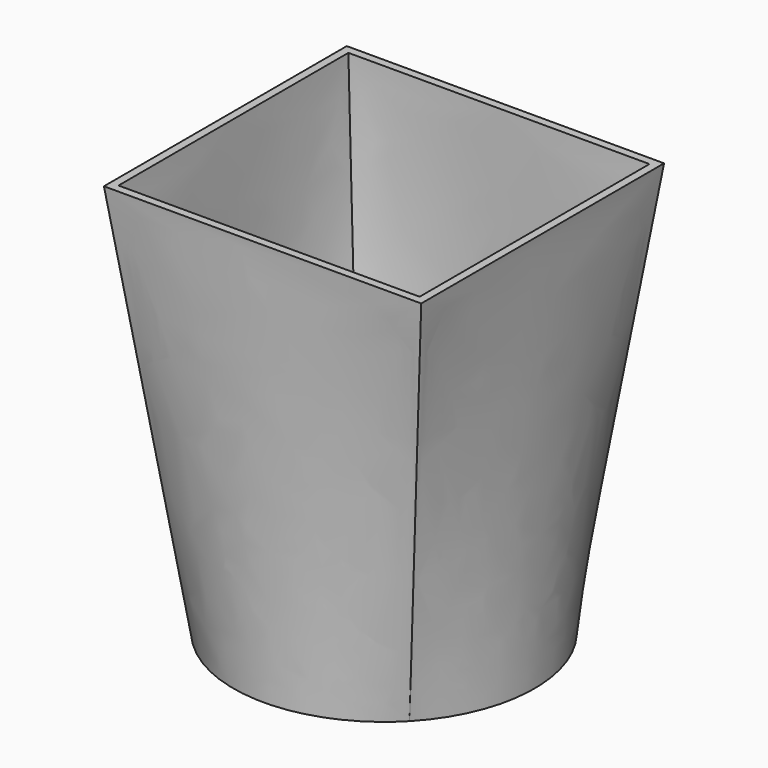
from build123d import *

# Parameters (mm, degrees)
F2_W = 99.9139621854
F2_H = 95.5784469843
F4_T = 2.54


# Not quite as in the source:
# - the arcs of a loft's sections are written as splines that run evenly, so that the points pair up as in the source's solid
# - a shell that OpenCascade refuses in one call is made with other operations: the cavity is built on its own and cut out


with BuildPart() as f3:
    # F2 (on offset) → F3 section 0
    with BuildSketch(Plane.XY.offset(127)):
        Rectangle(F2_W, F2_H)
    # F0 (on Top) → F3 section 1
    with BuildSketch(Plane.XY):
        with BuildLine():
            add(Edge.make_bspline(
                [(34.2488721695, -32.7627284648), (36.3931877331, -30.5211450231), (38.3166790346, -28.0684255821), (41.6482828465, -22.8347310657), (43.0563129764, -20.0538854036), (45.3028578067, -14.2707911992), (46.1413169567, -11.2686856553), (47.2164693474, -5.1584328302), (47.4531360028, -2.0504366369), (47.3155784505, 4.1521612197), (46.9413576443, 7.2466095116), (45.5963764086, 13.3031900424), (44.6256492365, 16.2651725205), (42.1249311921, 21.9429847323), (40.5950021549, 24.658674071), (37.0346484938, 29.7395228248), (35.0043119065, 32.1045566058), (32.7627284648, 34.2488721695)],
                knots=[0, 0, 0, 0, 0.125, 0.125, 0.25, 0.25, 0.375, 0.375, 0.5, 0.5, 0.625, 0.625, 0.75, 0.75, 0.875, 0.875, 1, 1, 1, 1], degree=3))
            add(Edge.make_bspline(
                [(32.7627284648, 34.2488721695), (30.5211450231, 36.3931877331), (28.0684255821, 38.3166790346), (22.8347310657, 41.6482828465), (20.0538854036, 43.0563129764), (14.2707911992, 45.3028578067), (11.2686856553, 46.1413169567), (5.1584328302, 47.2164693474), (2.0504366369, 47.4531360028), (-4.1521612197, 47.3155784505), (-7.2466095116, 46.9413576443), (-13.3031900424, 45.5963764086), (-16.2651725205, 44.6256492365), (-21.9429847323, 42.1249311921), (-24.658674071, 40.5950021549), (-29.7395228248, 37.0346484938), (-32.1045566058, 35.0043119065), (-34.2488721695, 32.7627284648)],
                knots=[0, 0, 0, 0, 0.125, 0.125, 0.25, 0.25, 0.375, 0.375, 0.5, 0.5, 0.625, 0.625, 0.75, 0.75, 0.875, 0.875, 1, 1, 1, 1], degree=3))
            add(Edge.make_bspline(
                [(-34.2488721695, 32.7627284648), (-36.3931877331, 30.5211450231), (-38.3166790346, 28.0684255821), (-41.6482828465, 22.8347310657), (-43.0563129764, 20.0538854036), (-45.3028578067, 14.2707911992), (-46.1413169567, 11.2686856553), (-47.2164693474, 5.1584328302), (-47.4531360028, 2.0504366369), (-47.3155784505, -4.1521612197), (-46.9413576443, -7.2466095116), (-45.5963764086, -13.3031900424), (-44.6256492365, -16.2651725205), (-42.1249311921, -21.9429847323), (-40.5950021549, -24.658674071), (-37.0346484938, -29.7395228248), (-35.0043119065, -32.1045566058), (-32.7627284648, -34.2488721695)],
                knots=[0, 0, 0, 0, 0.125, 0.125, 0.25, 0.25, 0.375, 0.375, 0.5, 0.5, 0.625, 0.625, 0.75, 0.75, 0.875, 0.875, 1, 1, 1, 1], degree=3))
            add(Edge.make_bspline(
                [(-32.7627284648, -34.2488721695), (-30.5211450231, -36.3931877331), (-28.0684255821, -38.3166790346), (-22.8347310657, -41.6482828465), (-20.0538854036, -43.0563129764), (-14.2707911992, -45.3028578067), (-11.2686856553, -46.1413169567), (-5.1584328302, -47.2164693474), (-2.0504366369, -47.4531360028), (4.1521612197, -47.3155784505), (7.2466095116, -46.9413576443), (13.3031900424, -45.5963764086), (16.2651725205, -44.6256492365), (21.9429847323, -42.1249311921), (24.658674071, -40.5950021549), (29.7395228248, -37.0346484938), (32.1045566058, -35.0043119065), (34.2488721695, -32.7627284648)],
                knots=[0, 0, 0, 0, 0.125, 0.125, 0.25, 0.25, 0.375, 0.375, 0.5, 0.5, 0.625, 0.625, 0.75, 0.75, 0.875, 0.875, 1, 1, 1, 1], degree=3))
        make_face()
    loft(ruled=True)

    # F4: shell of thickness 2.54, made by hand


with BuildPart() as f4_core1:
    # F4_t2: copy of F3
    add(f3.part)

    # the walls: a layer under each face that stays
    f4_faces = [f4_core1.faces().sort_by_distance(p)[0] for p in [
        (0.5254311457, -47.5867903594, 63.5),
        (48.6706691597, 0.5254311457, 63.5),
        (-0.5254311457, 47.5867903594, 63.5),
        (-48.6706691597, -0.5254311457, 63.5),
        (0, 0, 0),
    ]]
    thicken(f4_faces, amount=-F4_T, mode=Mode.SUBTRACT)


with BuildPart() as f3_1:
    add(f3.part)

    # what is left inside the walls is the cavity
    f4_cavity = [f4_core1.part.solids().sort_by_distance(p)[0] for p in [
        (0.329341, -45.091155, 85.374003),
    ]]
    add(f4_cavity, mode=Mode.SUBTRACT)


solid = f3_1.part
